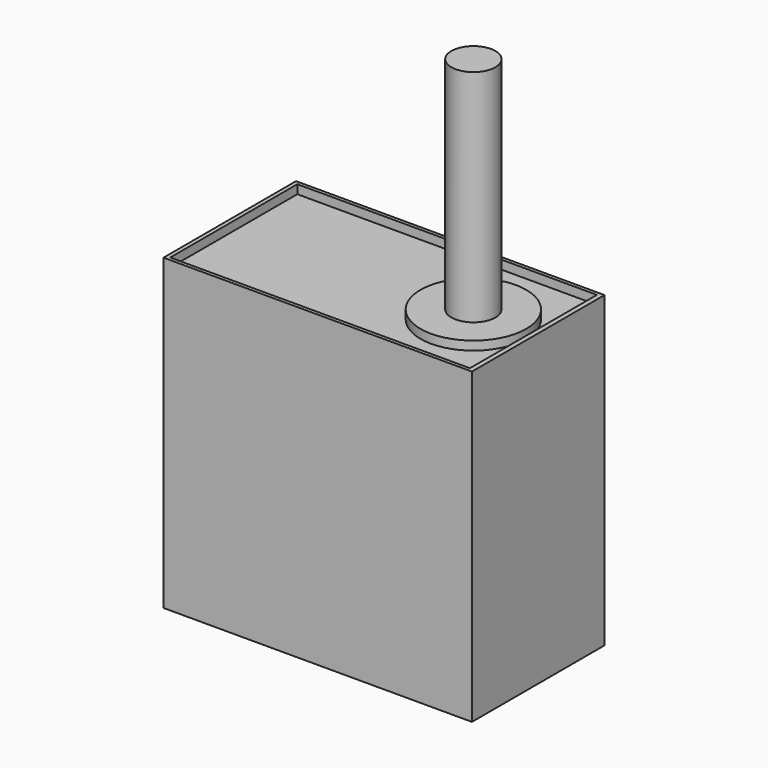
from build123d import *

# Parameters (mm, degrees)
F0_W     = 22.225
F0_H     = 11.938
F0_W_2   = 21.59
F0_H_2   = 11.4398148928
F1_DEPTH = 22.225
F0_R     = 3.81
F0_R_2   = 1.5875
F2_DEPTH = 22.225
F3_DEPTH = 38.1
F4_DEPTH = 21.59


with BuildPart() as f1:
    # F0 (on Top) → F1 (new body)
    with BuildSketch(Plane.XY):
        with Locations((-44.5170886815, 15.9408464691)):
            Rectangle(F0_W, F0_H)
        with Locations((-44.5462938675, 15.9408464691)):
            Rectangle(F0_W_2, F0_H_2, mode=Mode.SUBTRACT)
    extrude(amount=F1_DEPTH)



with BuildPart() as f2:
    # F0 (on Top) → F2 (new body)
    with BuildSketch(Plane.XY):
        with Locations((-38.077108562, 15.9408464691)):
            Circle(F0_R)
        with Locations((-38.077108562, 15.9408464691)):
            Circle(F0_R_2, mode=Mode.SUBTRACT)
    extrude(amount=F2_DEPTH)


with BuildPart() as f3:
    # F0 (on Top) → F3 (new body)
    with BuildSketch(Plane.XY):
        with Locations((-38.077108562, 15.9408464691)):
            Circle(F0_R_2)
    extrude(amount=F3_DEPTH)


with BuildPart() as f1_1:
    add(f1.part)

    add(f2.part)  # F4 merges F2
    # F0 (on Top) → F4 (join)
    with BuildSketch(Plane.XY):
        with Locations((-44.5170886815, 15.9408464691)):
            Rectangle(F0_W, F0_H)
        with Locations((-44.5462938675, 15.9408464691)):
            Rectangle(F0_W_2, F0_H_2, mode=Mode.SUBTRACT)
        with Locations((-44.5462938675, 15.9408464691)):
            Rectangle(F0_W_2, F0_H_2)
        with Locations((-38.077108562, 15.9408464691)):
            Circle(F0_R, mode=Mode.SUBTRACT)
    extrude(amount=F4_DEPTH)


solid = Compound([f3.part, f1_1.part])
